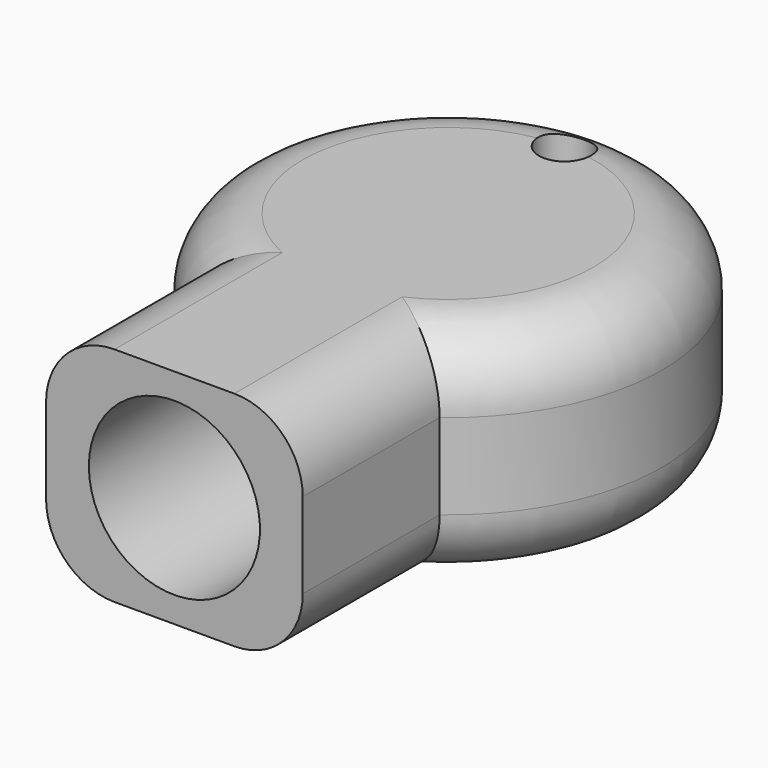
from build123d import *

# Parameters (mm, degrees)
F1_DEPTH = 16.51
F2_R     = 5.08
F4_D     = 3.81
F6_D     = 12.7
F6_DEPTH = 28.575
F6_TIP   = 3.8154649308


with BuildPart() as f1:
    # F0 (on Top) → F1 (new body)
    with BuildSketch(Plane.XY):
        with BuildLine():
            Line((9.525, -25.4), (9.525, -12.7))
            ThreePointArc((9.525, -12.7), (0, 15.875), (-9.525, -12.7))
            Line((-9.525, -12.7), (-9.525, -25.4))
            Line((-9.525, -25.4), (9.525, -25.4))
        make_face()
    extrude(amount=F1_DEPTH)

    # F2
    f2_edges = [f1.edges().sort_by_distance(p)[0] for p in [
        (0, 15.875, 16.51),
        (-9.525, -19.05, 16.51),
        (9.525, -19.05, 16.51),
        (0, 15.875, 0),
        (-9.525, -19.05, 0),
        (9.525, -19.05, 0),
    ]]
    fillet(f2_edges, radius=F2_R)

    # F4 (through all)
    with Locations(Plane.XY.offset(16.51)):
        with Locations((0, 10.795)):
            Hole(F4_D / 2)

    # F6
    with Locations(Plane.XZ.offset(25.4)):
        with Locations((0, 8.255)):
            Hole(F6_D / 2, depth=F6_DEPTH)
            with Locations((0, 0, -(F6_DEPTH + F6_TIP / 2))):  # 118° drill point
                Cone(0, F6_D / 2, F6_TIP, mode=Mode.SUBTRACT)


solid = f1.part
